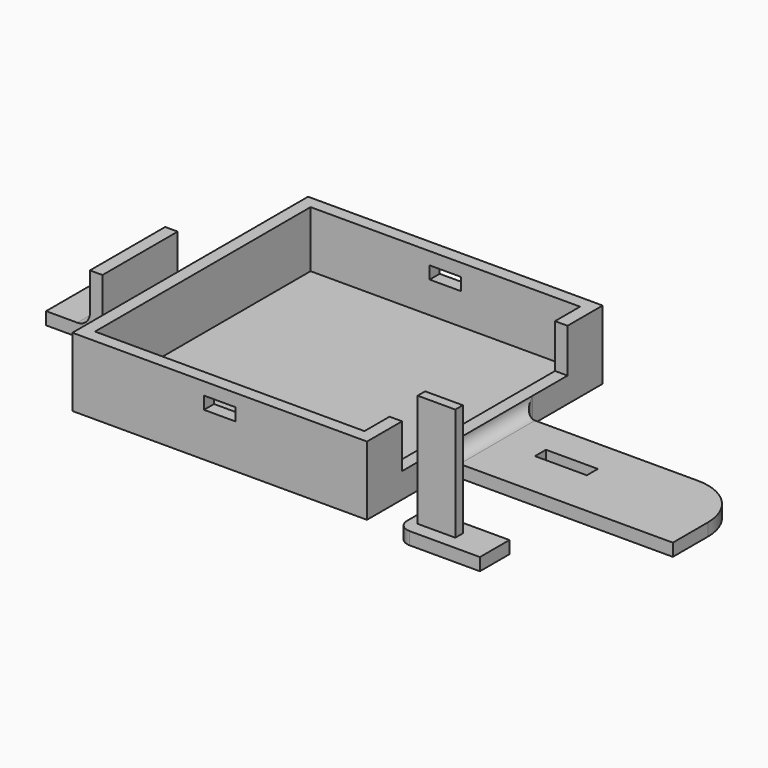
from build123d import *

# Parameters (mm, degrees)
F0_W      = 43
F0_H      = 43
F0_W_2    = 8
F0_H_2    = 13
F0_H_3    = 2
F0_W_3    = 7
F0_H_4    = 15
F1_DEPTH  = 2
F2_DEPTH  = 10
F3_DEPTH  = 11
F4_W      = 33
F4_H      = 7
F5_DEPTH  = 25
F6_R      = 1.99999
F7_DEPTH  = 25
F8_W      = 5
F8_H      = 2
F9_DEPTH  = 47.001
F10_W     = 6
F10_H     = 1.5
F11_DEPTH = 20
F12_DEPTH = 2


# Not quite as in the source:
# - a fillet or chamfer is up to 0.001 mm smaller than in the source, because OpenCascade refuses the exact size


with BuildPart() as f1:
    # F0 (on Top) → F1 (new body)
    with BuildSketch(Plane.XY):
        Polygon((23.5, -7.5), (40.5, -7.5), (59.5, -7.5), (59.5, -5.5), (36.5, -5.5), (23.5, -5.5), align=None)
        Polygon((23.5, -23.5), (23.5, -7.5), (23.5, -5.5), (23.5, 7.5), (23.5, 23.5), (-23.5, 23.5), (-23.5, 7.5), (-23.5, 5.5), (-23.5, -7.5), (-23.5, -23.5), align=None)
        Rectangle(F0_W, F0_H, mode=Mode.SUBTRACT)
        Polygon((23.5, 7.5), (23.5, -5.5), (36.5, -5.5), (36.5, 0), (31.5, 0), (31.5, 2.2), (36.5, 2.2), (36.5, 7.5), align=None)
        with BuildLine():
            Line((36.5, -5.5), (59.5, -5.5))
            Line((59.5, -5.5), (59.5, -0.5))
            ThreePointArc((59.5, -0.5), (57.1568542495, 5.1568542495), (51.5, 7.5))
            Line((51.5, 7.5), (40.5, 7.5))
            Line((40.5, 7.5), (36.5, 7.5))
            Line((36.5, 7.5), (36.5, 2.2))
            Line((36.5, 2.2), (39.7782735527, 2.2))
            Line((39.7782735527, 2.2), (39.7782735527, 0))
            Line((39.7782735527, 0), (36.5, 0))
            Line((36.5, 0), (36.5, -5.5))
        make_face()
        with Locations((-27.5, -1)):
            Rectangle(F0_W_2, F0_H_2)
        Polygon((-33.5, -7.5), (-31.5, -7.5), (-31.5, 5.5), (-31.5, 7.5), (-33.5, 7.5), align=None)
        with Locations((-27.5, 6.5)):
            Rectangle(F0_W_2, F0_H_3)
        with Locations((-37, 0)):
            Rectangle(F0_W_3, F0_H_4)
        Rectangle(F0_W, F0_H)
    extrude(amount=F1_DEPTH)

    # F0 (on Top) → F2 (join)
    with BuildSketch(Plane.XY):
        Polygon((-33.5, -7.5), (-31.5, -7.5), (-31.5, 5.5), (-31.5, 7.5), (-33.5, 7.5), align=None)
    extrude(amount=F2_DEPTH)

    # F0 (on Top) → F3 (join)
    with BuildSketch(Plane.XY):
        Polygon((23.5, -23.5), (23.5, -7.5), (23.5, -5.5), (23.5, 7.5), (23.5, 23.5), (-23.5, 23.5), (-23.5, 7.5), (-23.5, 5.5), (-23.5, -7.5), (-23.5, -23.5), align=None)
        Rectangle(F0_W, F0_H, mode=Mode.SUBTRACT)
    extrude(amount=F3_DEPTH)

    # F4 (on face) → F5 (cut)
    with BuildSketch(Plane.YZ.offset(23.5)):
        with Locations((0, 7.5)):
            Rectangle(F4_W, F4_H)
    extrude(amount=-F5_DEPTH, mode=Mode.SUBTRACT)

    # F6 (radius 2 in the source; OpenCascade refuses exactly that, so slightly less here)
    f6_edges = [f1.edges().sort_by_distance(p)[0] for p in [
        (-23.5, 0, 2),
        (-31.5, 0, 2),
        (23.5, 0, 2),
        (-33.5, 0, 2),
        (23.5, 7.5, 1),
        (-23.5, -7.5, 1),
        (23.5, -7.5, 1),
        (-23.5, 7.5, 1),
    ]]
    fillet(f6_edges, radius=F6_R)

    # F0 (on Top) → F7 (cut)
    with BuildSketch(Plane.XY):
        Polygon((31.5, 0), (36.5, 0), (39.7782735527, 0), (39.7782735527, 2.2), (36.5, 2.2), (31.5, 2.2), align=None)
    extrude(amount=-F7_DEPTH, mode=Mode.SUBTRACT)

    # F8 (on face) → F9 (cut, through all)
    with BuildSketch(Plane.XZ.offset(23.5)):
        with Locations((0, 8)):
            Rectangle(F8_W, F8_H)
    extrude(amount=-F9_DEPTH, mode=Mode.SUBTRACT)


with BuildPart() as f11:
    # F10 (on Top) → F11 (new body)
    with BuildSketch(Plane.XY):
        with Locations((34.5, -22.6426791698)):
            Rectangle(F10_W, F10_H)
    extrude(amount=F11_DEPTH)

    # F10 (on Top) → F12 (join)
    with BuildSketch(Plane.XY):
        with BuildLine():
            Line((43.161662899, -19.6656095535), (31.9530290067, -19.6656095535))
            ThreePointArc((31.9530290067, -19.6656095535), (30.5388154443, -20.2513959911), (29.9530290067, -21.6656095535))
            Line((29.9530290067, -21.6656095535), (29.9530290067, -23.5535977408))
            ThreePointArc((29.9530290067, -23.5535977408), (30.5388154443, -24.9678113032), (31.9530290067, -25.5535977408))
            Line((31.9530290067, -25.5535977408), (43.161662899, -25.5535977408))
            Line((43.161662899, -25.5535977408), (43.161662899, -19.6656095535))
        make_face()
        with Locations((34.5, -22.6426791698)):
            Rectangle(F10_W, F10_H, mode=Mode.SUBTRACT)
    extrude(amount=F12_DEPTH)


solid = Compound([f1.part, f11.part])
